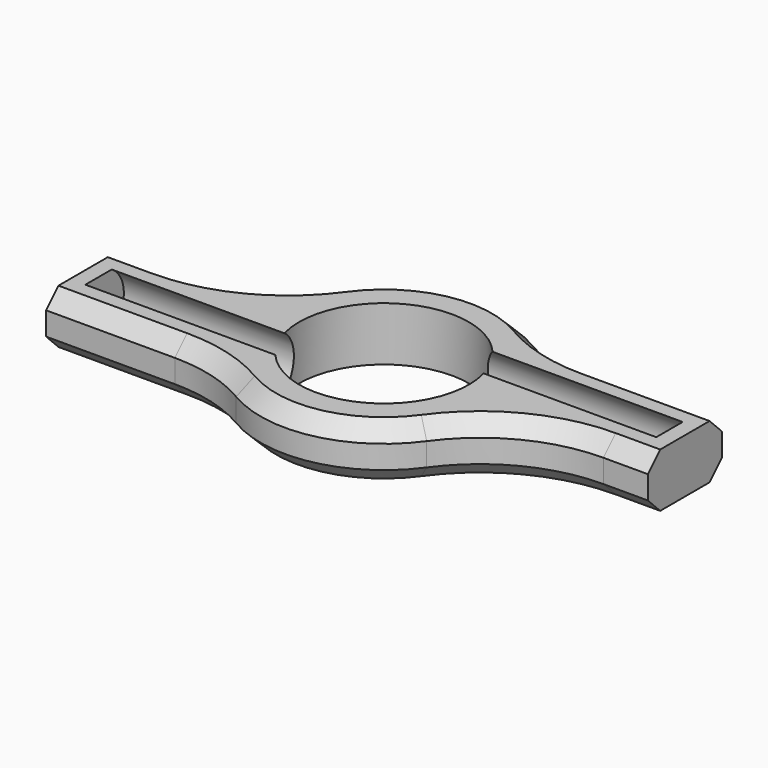
from build123d import *

# Parameters (mm, degrees)
F0_R     = 11
F1_DEPTH = 7
F2_R     = 4.1
F3_DEPTH = 28.8211942778
F4_R     = 4.1
F5_DEPTH = 28.8211942778
F6_W     = 12
F6_H     = 7
F7_DEPTH = 2
F8_W     = 12
F8_H     = 7
F9_DEPTH = 2
F10_R    = 20
F11_SIZE = 2


# Not quite as in the source:
# - a feature names something its author has since deleted; it is built from what else it names


with BuildPart() as f1:
    # F0 (on Top) → F1 (new body)
    with BuildSketch(Plane.XY):
        with BuildLine():
            Line((35, 11), (11.6189500386, 11))
            ThreePointArc((11.6189500386, 11), (-5.4525336701, 15.0422696617), (-15.9687194227, 1))
            Line((-15.9687194227, 1), (-35, 1))
            Line((-35, 1), (-35, -11))
            Line((-35, -11), (-11.6189500386, -11))
            ThreePointArc((-11.6189500386, -11), (5.4525336701, -15.0422696617), (15.9687194227, -1))
            Line((15.9687194227, -1), (35, -1))
            Line((35, -1), (35, 11))
        make_face()
        Circle(F0_R, mode=Mode.SUBTRACT)
    extrude(amount=F1_DEPTH)

    # F2 (on face) → F3 (cut, through all)
    with BuildSketch(Plane.YZ.offset(35)):
        with Locations((5, 3.5)):
            Circle(F2_R)
    extrude(amount=-F3_DEPTH, mode=Mode.SUBTRACT)

    # F4 (on face) → F5 (cut, through all)
    with BuildSketch(Plane(origin=(-35, 0, 0), x_dir=(0, -1, 0), z_dir=(-1, 0, 0))):
        with Locations((5, 3.5)):
            Circle(F4_R)
    extrude(amount=-F5_DEPTH, mode=Mode.SUBTRACT)

    # F6 (on face) → F7 (join)
    with BuildSketch(Plane.YZ.offset(35)):
        with Locations((5, 3.5)):
            Rectangle(F6_W, F6_H)
    extrude(amount=-F7_DEPTH)

    # F8 (on face) → F9 (join)
    with BuildSketch(Plane(origin=(-35, 0, 0), x_dir=(0, -1, 0), z_dir=(-1, 0, 0))):
        with Locations((5, 3.5)):
            Rectangle(F8_W, F8_H)
    extrude(amount=-F9_DEPTH)

    # F10
    f10_edges = [f1.edges().sort_by_distance(p)[0] for p in [
        (11.61895, 11, 3.5),
        (-15.968719, 1, 3.5),
        (15.968719, -1, 3.5),
        (-11.61895, -11, 3.5),
    ]]
    fillet(f10_edges, radius=F10_R)

    # F11
    f11_edges = [f1.edges().sort_by_distance(p)[0] for p in [
        (-26.651503, -11, 7),
        (32.120192, -1, 7),
        (-3.293287, 15.657403, 7),
        (-32.120192, 1, 7),
        (32.120192, -1, 0),
        (-3.293287, 15.657403, 0),
        (-26.651503, -11, 0),
        (-32.120192, 1, 0),
    ]]
    chamfer(f11_edges, length=F11_SIZE)


solid = f1.part
